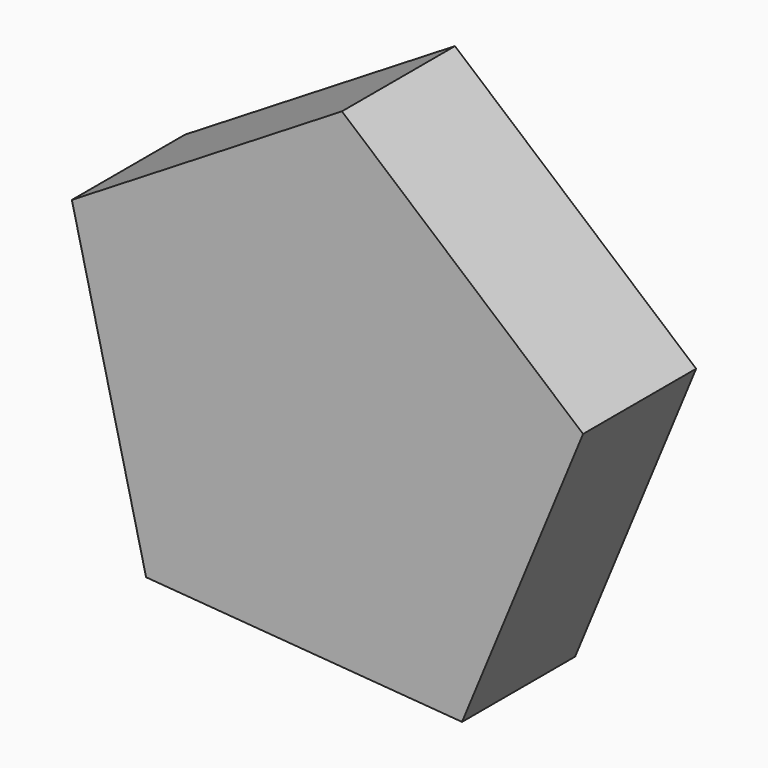
from build123d import *

# Parameters (mm, degrees)
F3_DEPTH = 25.4
F4_T     = -2.54


# Not quite as in the source:
# - the program builds the solid bodies; features that only make, move or delete a surface that nothing else refers to are left out


with BuildPart() as f3:
    # F2 (on Front) → F3 (new body)
    with BuildSketch(Plane.XZ):
        Polygon((3.7617208479, 48.2991386944), (-44.7727749167, 18.5028637951), (-31.4328175171, -36.8637399798), (25.346225329, -41.2859080551), (47.0976462569, 11.3476455454), align=None)
    extrude(amount=F3_DEPTH)

    # F4
    f4_openings = [f3.faces().sort_by_distance(p)[0] for p in [
        (0, 0, 0),
    ]]
    offset(amount=F4_T, openings=f4_openings)


solid = f3.part
